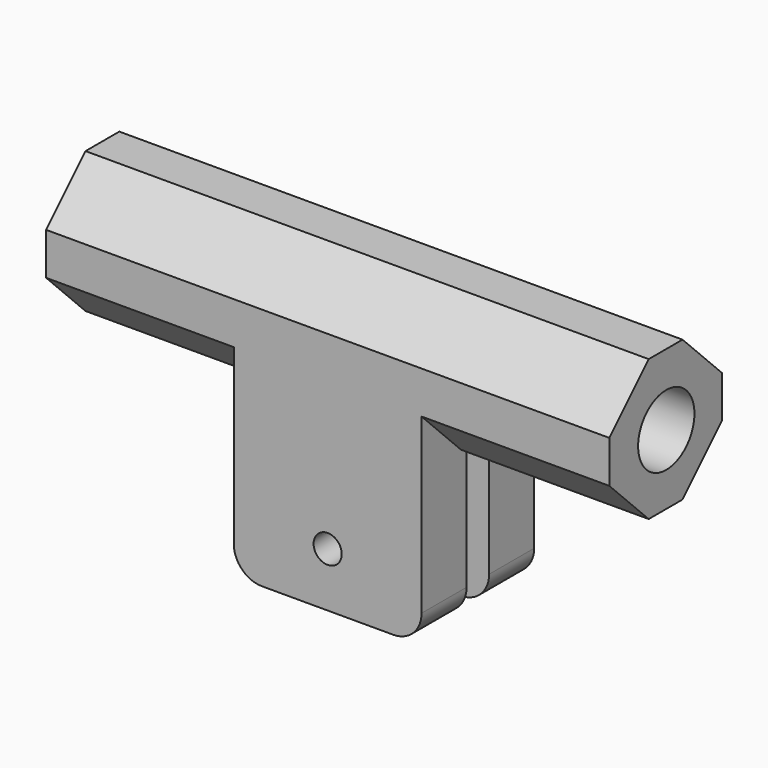
from build123d import *

# Parameters (mm, degrees)
F1_DEPTH = 6.35
F0_W     = 8.4666666667
F0_H     = 6.858
F2_DEPTH = 6.35
F3_SIZE  = 2.2225
F4_R     = 1.27
F5_T     = 2.54
F7_D     = 3.175
F7_DEPTH = 25.4
F7_TIP   = 0.9538662327
F9_D     = 1.27
F9_DEPTH = 25.4
F9_TIP   = 0.3815464931


# Not quite as in the source:
# - a shell that OpenCascade refuses in one call is made with other operations: the cavity is built on its own and cut out


with BuildPart() as f1:
    # F0 (on Front) → F1 (new body)
    with BuildSketch(Plane.XZ):
        Polygon((12.7, -3.175), (12.7, 3.175), (-12.7, 3.175), (-12.7, -3.175), (-4.2333333333, -3.175), (4.2333333333, -3.175), align=None)
    extrude(amount=F1_DEPTH)

    # F0 (on Front) → F2 (join)
    with BuildSketch(Plane.XZ):
        with Locations((0, -6.604)):
            Rectangle(F0_W, F0_H)
    extrude(amount=F2_DEPTH)

    # F3
    f3_edges = [f1.edges().sort_by_distance(p)[0] for p in [
        (0, -6.35, 3.175),
        (8.466667, -6.35, -3.175),
        (-8.466667, -6.35, -3.175),
        (0, 0, 3.175),
        (8.466667, 0, -3.175),
        (-8.466667, 0, -3.175),
    ]]
    chamfer(f3_edges, length=F3_SIZE)

    # F4
    f4_edges = [f1.edges().sort_by_distance(p)[0] for p in [
        (-4.233333, -3.175, -10.033),
        (4.233333, -3.175, -10.033),
    ]]
    fillet(f4_edges, radius=F4_R)

    # F5: shell of thickness 2.54, made by hand


with BuildPart() as f5_core1:
    # F5_t2: copy of F1
    add(f1.part)

    # the walls: a layer under each face that stays
    f5_faces = [f5_core1.faces().sort_by_distance(p)[0] for p in [
        (0, 0, -4.54025),
        (8.4666666667, -1.11125, -2.06375),
        (12.7, -3.175, 0),
        (0, -1.11125, 2.06375),
        (-12.7, -3.175, 0),
        (-8.4666666667, -1.11125, -2.06375),
        (0, -6.35, -4.54025),
        (8.4666666667, -3.175, -3.175),
        (8.4666666667, -5.23875, -2.06375),
        (0, -5.23875, 2.06375),
        (0, -3.175, 3.175),
        (-8.4666666667, -3.175, -3.175),
        (-8.4666666667, -5.23875, -2.06375),
    ]]
    thicken(f5_faces, amount=-F5_T, mode=Mode.SUBTRACT)


with BuildPart() as f1_1:
    add(f1.part)

    # what is left inside the walls is the cavity
    f5_cavity = [f5_core1.part.solids().sort_by_distance(p)[0] for p in [
        (0, -2.5654, -6.721867),
    ]]
    add(f5_cavity, mode=Mode.SUBTRACT)

    # F7
    with Locations(Plane(origin=(-12.7, 0, 0), x_dir=(0, -1, 0), z_dir=(-1, 0, 0))):
        with Locations((3.1371232575, -0.0378767425)):
            Hole(F7_D / 2, depth=F7_DEPTH)
            with Locations((0, 0, -(F7_DEPTH + F7_TIP / 2))):  # 118° drill point
                Cone(0, F7_D / 2, F7_TIP, mode=Mode.SUBTRACT)

    # F9
    with Locations(Plane.XZ.offset(6.35)):
        with Locations((0, -7.5871711597)):
            Hole(F9_D / 2, depth=F9_DEPTH)
            with Locations((0, 0, -(F9_DEPTH + F9_TIP / 2))):  # 118° drill point
                Cone(0, F9_D / 2, F9_TIP, mode=Mode.SUBTRACT)


solid = f1_1.part
